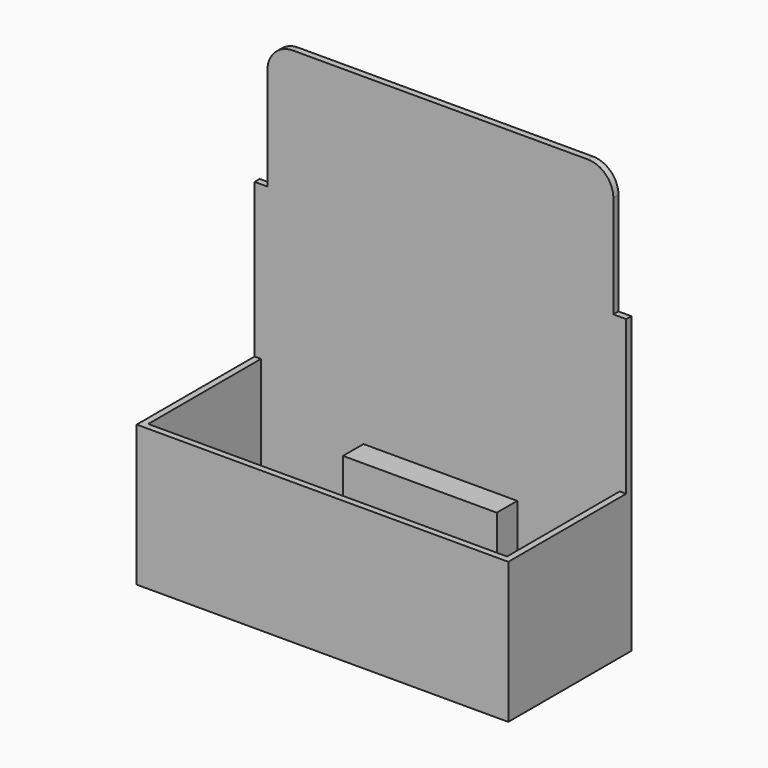
from build123d import *

# Parameters (mm, degrees)
F0_W          = 184.15
F0_H          = 76.2
F1_DEPTH      = 3.175
F2_W          = 177.8
F2_H          = 3.1757424533
F3_DEPTH      = 66.675
F4_W          = 184.15
F4_H          = 3.1757424533
F5_DEPTH      = 76.2
F6_W          = 171.4427173138
F6_H          = 3.1757424533
F7_DEPTH      = 63.5
F8_R          = 12.7
F9_W          = 76.2
F9_H          = 25.4
F10_DEPTH     = 12.7
F12_DEPTH     = 0.254
F13_TEXT_SIZE = 24.4062497384
F14_DEPTH     = 0.254


# Not quite as in the source:
# - Text() gives the source's letters only with a copy of the font that has no kerning and outlines rounded to 1/6400 em; it was checked with that copy


with BuildPart() as f1:
    # F0 (on Top) → F1 (new body)
    with BuildSketch(Plane.XY):
        Rectangle(F0_W, F0_H)
    extrude(amount=F1_DEPTH)

    # F2 (on face) → F3 (join)
    with BuildSketch(Plane.XY.offset(3.175)):
        Polygon((-88.9, 38.1), (-92.075, 38.1), (-92.075, -38.1), (-88.9, -38.1), (-88.9, -34.9242575467), (-88.9, 34.9242575467), align=None)
        with Locations((0, 36.5121287733)):
            Rectangle(F2_W, F2_H)
        Polygon((92.075, 38.1), (88.9, 38.1), (88.9, 34.9242575467), (88.9, -34.9242575467), (88.9, -38.1), (92.075, -38.1), align=None)
        with Locations((0, -36.5121287733)):
            Rectangle(F2_W, F2_H)
    extrude(amount=F3_DEPTH)

    # F4 (on face) → F5 (join)
    with BuildSketch(Plane.XY.offset(69.85)):
        with Locations((0, 36.5121287733)):
            Rectangle(F4_W, F4_H)
    extrude(amount=F5_DEPTH)

    # F6 (on face) → F7 (join)
    with BuildSketch(Plane.XY.offset(146.05)):
        with Locations((0.0007376075, 36.5121287733)):
            Rectangle(F6_W, F6_H)
    extrude(amount=F7_DEPTH)

    # F8
    f8_edges = [f1.edges().sort_by_distance(p)[0] for p in [
        (-85.720621, 36.512129, 209.55),
        (85.722096, 36.512129, 209.55),
    ]]
    fillet(f8_edges, radius=F8_R)

    # F9 (on face) → F10 (join)
    with BuildSketch(Plane.XZ.offset(-34.9242575467)):
        with Locations((0, 36.5125)):
            Rectangle(F9_W, F9_H)
    extrude(amount=F10_DEPTH)

    # F11 (on face) → F12 (join)
    with BuildSketch(Plane(origin=(0, 38.1, 0), x_dir=(-1, 0, 0), z_dir=(0, 1, 0))):
        Polygon((-50.8003688037, 82.6732463842), (-0.0001221367, 82.6732463842), (-0.0006154708, 133.4732463842), (-50.8003688037, 133.4732463842), align=None)
        Polygon((-0.0006154708, 133.4732463842), (-0.0001221367, 82.6732463842), (50.7996311963, 82.6732463842), (50.7996311963, 133.4732463842), align=None)
    extrude(amount=F12_DEPTH)

    # F13 (on face) → F14 (join)
    with BuildSketch(Plane(origin=(0, 38.354, 0), x_dir=(-1, 0, 0), z_dir=(0, 1, 0))):
        with Locations(Location((36.7524203094, 116.9829890132), (0, 0, -180))):
            Text('LABEL', F13_TEXT_SIZE, font='Open Sans', text_align=(TextAlign.LEFT, TextAlign.BOTTOM))
    extrude(amount=F14_DEPTH)


solid = f1.part
